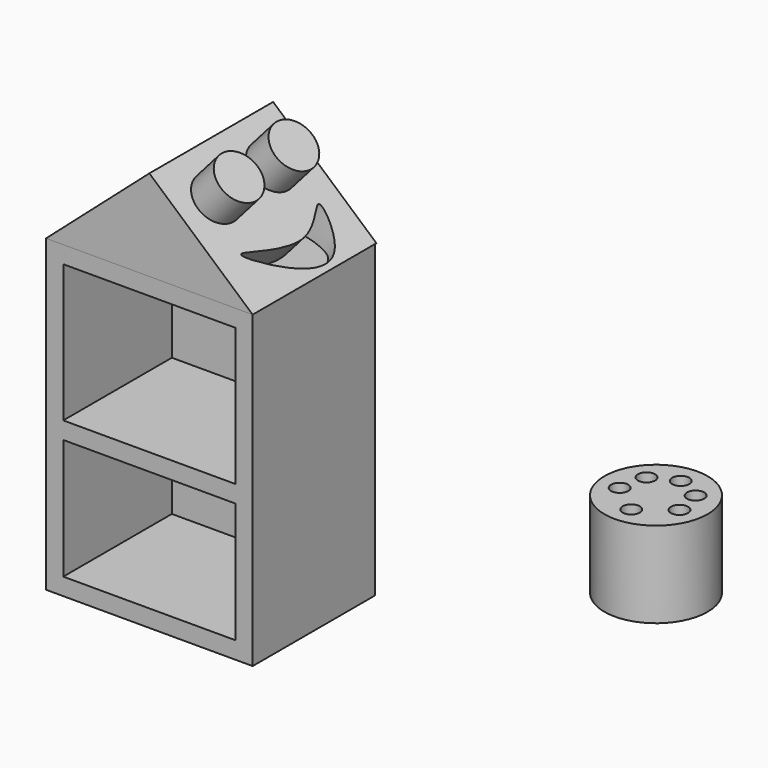
from build123d import *

# Parameters (mm, degrees)
F0_R      = 15
F1_DEPTH  = 25
F2_R      = 2.5
F3_DEPTH  = 25
F4_W      = 60.0831918418
F4_H      = 44.4846190512
F5_DEPTH  = 45
F6_T      = -5
F7_W      = 60.0831918418
F7_H      = 44.4846190512
F8_DEPTH  = 45
F9_T      = -5
F11_DEPTH = 45
F12_R     = 6.7226882027
F13_DEPTH = 10
F15_DEPTH = 10


# Not quite as in the source:
# - a shell that OpenCascade refuses in one call is made with other operations: the cavity is built on its own and cut out


with BuildPart() as f1:
    # F0 (on Top) → F1 (new body)
    with BuildSketch(Plane.XY):
        Circle(F0_R)
    extrude(amount=F1_DEPTH)

    # F2 (on face) → F3 (cut)
    with BuildSketch(Plane.XY.offset(25)):
        with Locations((0, 9)):
            Circle(F2_R)
        with Locations((7.1401800626, 5.4788528611)):
            Circle(F2_R)
        with Locations((8.6933324366, -2.3293714059)):
            Circle(F2_R)
        with Locations((0, -9)):
            Circle(F2_R)
        with Locations((-8.6933324366, -2.3293714059)):
            Circle(F2_R)
        with Locations((-7.1401800626, 5.4788528611)):
            Circle(F2_R)
    extrude(amount=-F3_DEPTH, mode=Mode.SUBTRACT)


with BuildPart() as f5:
    # F4 (on Top) → F5 (new body)
    with BuildSketch(Plane.XY):
        with Locations((-79.0518615395, -63.140777871)):
            Rectangle(F4_W, F4_H)
    extrude(amount=F5_DEPTH)

    # F6
    f6_openings = [f5.faces().sort_by_distance(p)[0] for p in [
        (-79.051862, -85.383087, 22.5),
    ]]
    offset(amount=F6_T, openings=f6_openings)

    # F7 (on face) → F8 (join)
    with BuildSketch(Plane.XY.offset(45)):
        with Locations((-79.0518615395, -63.140777871)):
            Rectangle(F7_W, F7_H)
    extrude(amount=F8_DEPTH)

    # F9: a shell. OpenCascade refuses it in one call, so the cavity is built on its own and cut out:
    # the body offset inwards by the wall thickness, plus a prism from it out through each open face.
    f9_core = offset(f5.part, amount=F9_T, kind=Kind.INTERSECTION, mode=Mode.PRIVATE)
    f9_exits = [f9_core.faces().sort_by_distance(p)[0] for p in [
        (-79.051862, -80.383087, 65),
    ]]
    add(f9_core, mode=Mode.SUBTRACT)
    extrude(f9_exits, amount=-F9_T, mode=Mode.SUBTRACT)


with BuildPart() as f11:
    # F10 (on face) → F11 (new body)
    with BuildSketch(Plane.XZ.offset(85.3830873966)):
        Polygon((-79.0518615395, 116.4102728976), (-109.0934574604, 90), (-49.0102656186, 90), align=None)
    extrude(amount=-F11_DEPTH)

    # F12 (on face) → F13 (join)
    with BuildSketch(Plane(origin=(23.2636398019, 0, 26.462311438), x_dir=(0.751039898, 0, -0.6602568224), z_dir=(0.6602568224, 0, 0.751039898))):
        with Locations((-123.6231103539, -72.8490576148)):
            Circle(F12_R)
        with Locations((-123.6231103539, -52.9171171784)):
            Circle(F12_R)
    extrude(amount=F13_DEPTH)

    # F14 (on face) → F15 (cut)
    with BuildSketch(Plane(origin=(23.2636398019, 0, 26.462311438), x_dir=(0.751039898, 0, -0.6602568224), z_dir=(0.6602568224, 0, 0.751039898))):
        with BuildLine():
            add(Edge.make_bspline(
                [(-109.5984280109, -76.9930705428), (-110.1601459247, -75.784375773), (-100.1559948089, -57.042503909), (-116.4868054447, -44.7783872856), (-94.301212557, -51.2157540048), (-100.3186965693, -67.9573528502), (-109.1734075078, -77.9076222184), (-109.5984280109, -76.9930705428)],
                knots=[0, 0, 0, 0, 0.2378158667, 0.4175512932, 0.6025298613, 0.8200580454, 1, 1, 1, 1], degree=3))
        make_face()
    extrude(amount=-F15_DEPTH, mode=Mode.SUBTRACT)


solid = Compound([f1.part, f5.part, f11.part])
